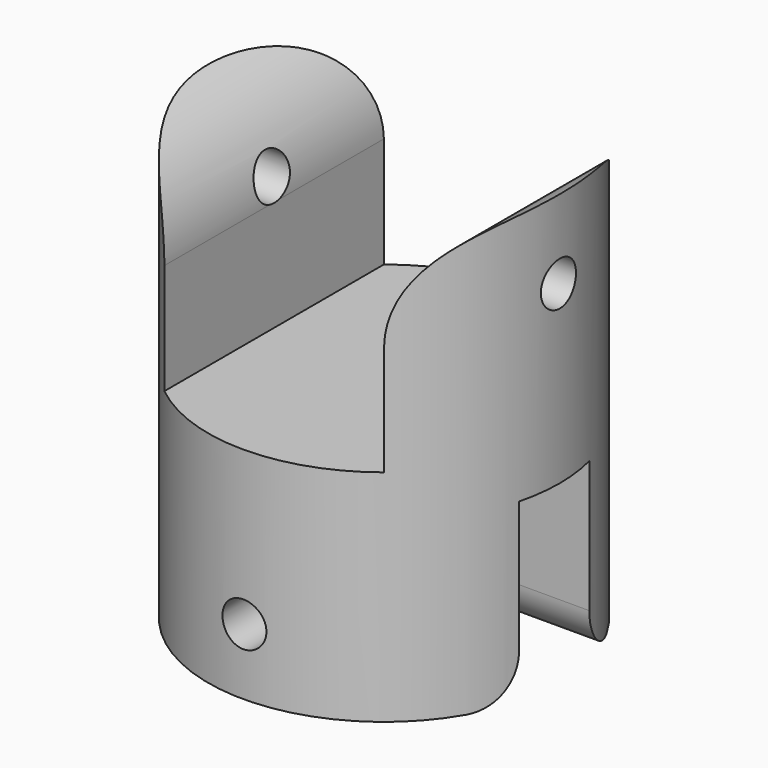
from build123d import *

# Parameters (mm, degrees)
F0_R        = 8
F1_DEPTH    = 10
F3_DEPTH    = 10
F5_D        = 2
F5_DEPTH    = 8.001
F6_D        = 2
F7_T1_DEPTH = 37.4894960018
F9_DEPTH    = 8
F11_D       = 2
F11_DEPTH   = 8.0010001
F13_D       = 2
F14_R       = 1.99999


# Not quite as in the source:
# - a fillet or chamfer that OpenCascade refuses, or shapes differently, is made with other operations: its cross-section is extruded or revolved along the edge and cut away or added
# - a fillet or chamfer is up to 0.001 mm smaller than in the source, because OpenCascade refuses the exact size


with BuildPart() as f1:
    # F0 (on Top) → F1 (new body, symmetric)
    with BuildSketch(Plane.XY):
        Circle(F0_R)
    extrude(amount=F1_DEPTH, both=True)

    # F2 (on face) → F3 (cut)
    with BuildSketch(Plane.XY.offset(10)):
        with BuildLine():
            ThreePointArc((5, 6.2449979984), (0, 8), (-5, 6.2449979984))
            Line((-5, 6.2449979984), (-5, -6.2449979984))
            ThreePointArc((-5, -6.2449979984), (0, -8), (5, -6.2449979984))
            Line((5, -6.2449979984), (5, 6.2449979984))
        make_face()
    extrude(amount=-F3_DEPTH, mode=Mode.SUBTRACT)

    # F5 (through all, one way)
    with BuildSketch(Plane.YZ):
        with Locations((0, 6)):
            Circle(F5_D / 2)
    extrude(amount=-F5_DEPTH, mode=Mode.SUBTRACT)

    # F6 (through all)
    with Locations(Plane(origin=(0, 0, 0), x_dir=(0, 1, 0), z_dir=(-1, 0, 0))):
        with Locations((0, -6)):
            Hole(F6_D / 2)

    # F7: fillet of radius 5 on 2 edges, made by hand

    # F7_s2 → F7_t1 (cut)
    with BuildSketch(Plane.XZ.offset(-18.7447480009)):
        with BuildLine():
            ThreePointArc((-4.9999, 5.0001), (-6.4643660941, 8.5356339059), (-9.9999, 10.0001))
            Line((-9.9999, 10.0001), (-9.9999, 10.1001))
            ThreePointArc((-9.9999, 10.1001), (-7.49995, 10.1), (-5, 10.1))
            Line((-5, 10.1), (-4.9, 10))
            ThreePointArc((-4.9, 10), (-4.9, 7.50005), (-4.8999, 5.0001))
            Line((-4.8999, 5.0001), (-4.9999, 5.0001))
        make_face()
        with BuildLine():
            ThreePointArc((9.9999, 10.0001), (6.4643660941, 8.5356339059), (4.9999, 5.0001))
            Line((4.9999, 5.0001), (4.8999, 5.0001))
            ThreePointArc((4.8999, 5.0001), (4.9, 7.50005), (4.9, 10))
            Line((4.9, 10), (5, 10.1))
            ThreePointArc((5, 10.1), (7.49995, 10.1), (9.9999, 10.1001))
            Line((9.9999, 10.1001), (9.9999, 10.0001))
        make_face()
    extrude(amount=F7_T1_DEPTH, mode=Mode.SUBTRACT)

    # F8 (on face) → F9 (cut)
    with BuildSketch(Plane(origin=(0, 0, -10), x_dir=(1, 0, 0), z_dir=(0, 0, -1))):
        with BuildLine():
            Line((7.7459666924, 2), (-7.7459666924, 2))
            ThreePointArc((-7.7459666924, 2), (-8, 0), (-7.7459666924, -2))
            Line((-7.7459666924, -2), (7.7459666924, -2))
            ThreePointArc((7.7459666924, -2), (7.9362375701, -1.0080343399), (8, 0))
            ThreePointArc((8, 0), (7.9362375701, 1.0080343399), (7.7459666924, 2))
        make_face()
    extrude(amount=-F9_DEPTH, mode=Mode.SUBTRACT)

    # F11 (through all, one way)
    with BuildSketch(Plane.XZ):
        with Locations((0, -7)):
            Circle(F11_D / 2)
    extrude(amount=-F11_DEPTH, mode=Mode.SUBTRACT)

    # F13 (through all)
    with Locations(Plane(origin=(0, 0, 0), x_dir=(1, 0, 0), z_dir=(0, 1, 0))):
        with Locations((0, 7)):
            Hole(F13_D / 2)

    # F14 (radius 2 in the source; OpenCascade refuses exactly that, so slightly less here)
    f14_edges = [f1.edges().sort_by_distance(p)[0] for p in [
        (0, -2, -10),
        (0, 2, -10),
    ]]
    fillet(f14_edges, radius=F14_R)


solid = f1.part
